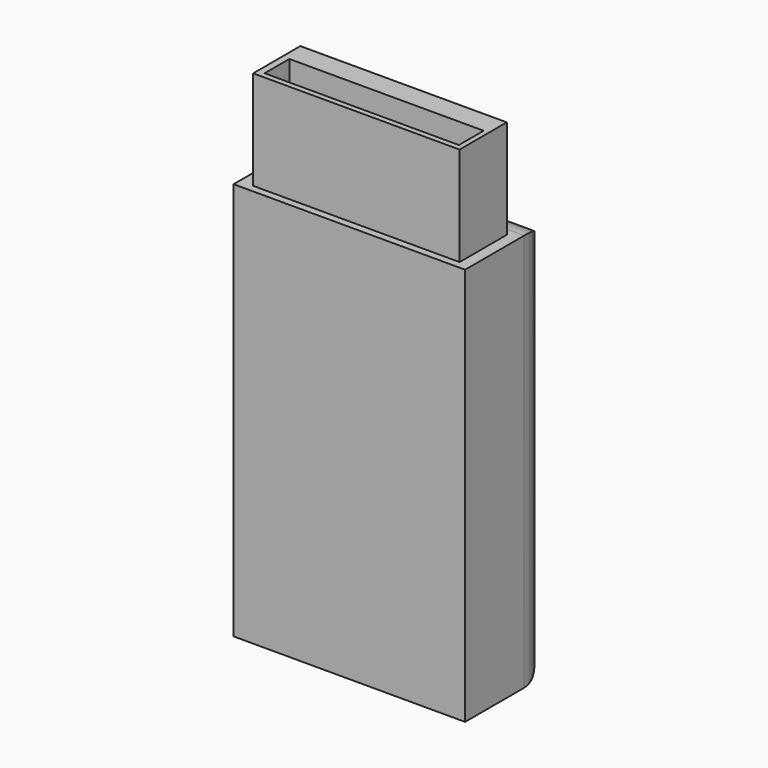
from build123d import *

# Parameters (mm, degrees)
F0_W        = 15.7
F0_H        = 27
F1_DEPTH    = 7.5
F2_W        = 14
F2_H        = 18.5080650263
F3_DEPTH    = 4
F7_T1_DEPTH = 28.2
F7_T3_DEPTH = 39.5
F8_W        = 13.1793060163
F8_H        = 2.1
F9_DEPTH    = 7.5


# Not quite as in the source:
# - a fillet or chamfer that OpenCascade refuses, or shapes differently, is made with other operations: its cross-section is extruded or revolved along the edge and cut away or added


with BuildPart() as f1:
    # F0 (on Front) → F1 (new body)
    with BuildSketch(Plane.XZ):
        with Locations((-45.7689563572, 18.127016373)):
            Rectangle(F0_W, F0_H)
    extrude(amount=F1_DEPTH)


with BuildPart() as f3:
    # F2 (on Front) → F3 (new body)
    with BuildSketch(Plane.XZ):
        with Locations((-45.8931468725, -4.8084680457)):
            Rectangle(F2_W, F2_H)
    extrude(amount=F3_DEPTH)


with BuildPart() as f3_1:
    # F4: moved
    add(f3.part.moved(Location((0.2, -0.9, 15.2))))


with BuildPart() as f1_1:
    add(f1.part)

    # F5: cut F3
    add(f3_1.part, mode=Mode.SUBTRACT)

    # F7: fillet of radius 2.5 on 4 edges, made by hand

    # F7_s2 → F7_t1 (cut)
    with BuildSketch(Plane.YZ.offset(-59.8689563572)):
        with BuildLine():
            ThreePointArc((-2.5, 31.627016373), (-0.732233047, 30.8947833259), (0, 29.127016373))
            Line((0, 29.127016373), (0, 31.627016373))
            Line((0, 31.627016373), (-2.5, 31.627016373))
        make_face()
        with BuildLine():
            ThreePointArc((0, 7.127016373), (-0.732233047, 5.35924942), (-2.5, 4.627016373))
            Line((-2.5, 4.627016373), (0, 4.627016373))
            Line((0, 4.627016373), (0, 7.127016373))
        make_face()
    extrude(amount=F7_T1_DEPTH, mode=Mode.SUBTRACT)

    # F7_s4 → F7_t3 (cut)
    with BuildSketch(Plane.XY.offset(-1.622983627)):
        with BuildLine():
            ThreePointArc((-53.6189563572, -2.5), (-52.8867233102, -0.732233047), (-51.1189563572, 0))
            Line((-51.1189563572, 0), (-53.6189563572, 0))
            Line((-53.6189563572, 0), (-53.6189563572, -2.5))
        make_face()
        with BuildLine():
            ThreePointArc((-37.9189563572, -2.5), (-38.6511894043, -0.732233047), (-40.4189563572, 0))
            Line((-40.4189563572, 0), (-37.9189563572, 0))
            Line((-37.9189563572, 0), (-37.9189563572, -2.5))
        make_face()
    extrude(amount=F7_T3_DEPTH, mode=Mode.SUBTRACT)


with BuildPart() as f3_2:
    # F6: moved
    add(f3_1.part.moved(Location((0, -2.1, 18.7))))


with BuildPart() as f9:
    # F8 (on Top) → F9 (new body)
    with BuildSketch(Plane.XY):
        with Locations((-45.6346645951, -5.5668568239)):
            Rectangle(F8_W, F8_H)
    extrude(amount=F9_DEPTH)


with BuildPart() as f9_1:
    # F10: moved
    add(f9.part.moved(Location((0, 0, 35.9))))


with BuildPart() as f3_3:
    add(f3_2.part)

    # F11: cut F9
    add(f9_1.part, mode=Mode.SUBTRACT)


solid = Compound([f1_1.part, f3_3.part])
